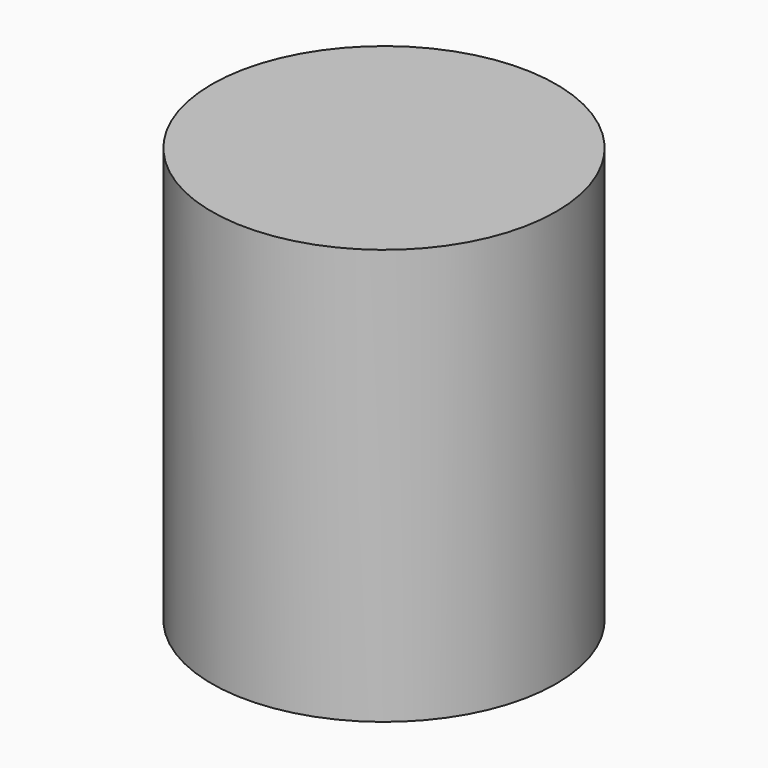
from build123d import *

# Parameters (mm, degrees)
F0_R     = 49.8119977907
F1_DEPTH = 120.142


# Not quite as in the source:
# - a feature of the source that left no trace in its solid (it failed there, or was rolled back) is left out


with BuildPart() as f1:
    # F0 (on Top) → F1 (new body)
    with BuildSketch(Plane.XY):
        Circle(F0_R)
    extrude(amount=F1_DEPTH)


solid = f1.part
